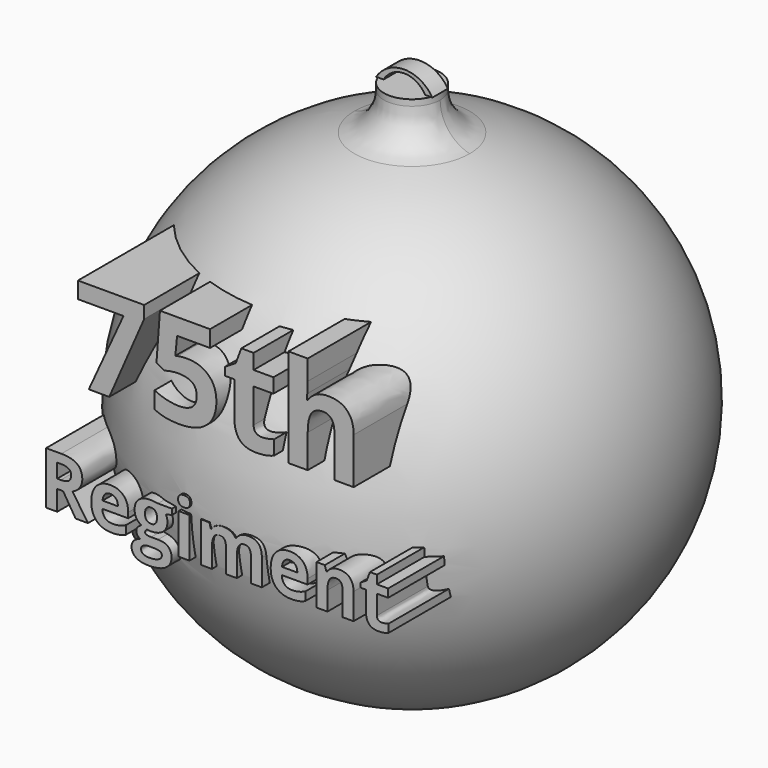
from build123d import *

# Parameters (mm, degrees)
F2_R          = 3.6879360159
F3_DEPTH      = 36.576
F4_R          = 5.08
F6_DEPTH      = 1.27
F8_DEPTH      = 12.7
F9_TEXT_SIZE  = 16.9737471475
F10_DEPTH     = 31.242
F11_TEXT_SIZE = 9.6334003123
F12_DEPTH     = 31.75


# Not quite as in the source:
# - Text() gives the source's letters only with a copy of the font that has no kerning and outlines rounded to 1/6400 em; it was checked with that copy


with BuildPart() as f1:
    # F0 (on Front) → F1 (revolve)
    with BuildSketch(Plane.XZ):
        with BuildLine():
            Line((0, -31.75), (0, 31.75))
            ThreePointArc((0, 31.75), (-31.75, 0), (0, -31.75))
        make_face()
    revolve(axis=Axis((0, 0, -12.3165734112), (0, 0, -1)))

    # F2 (on Top) → F3 (join)
    with BuildSketch(Plane.XY):
        Circle(F2_R)
    extrude(amount=F3_DEPTH)

    # F4
    f4_edges = [f1.edges().sort_by_distance(p)[0] for p in [
        (0, -3.687936, 31.535086),
        (0, 3.687936, 31.535086),
    ]]
    fillet(f4_edges, radius=F4_R)

    # F5 (on Front) → F6 (join, symmetric)
    with BuildSketch(Plane.XZ):
        with BuildLine():
            ThreePointArc((3.6879360159, 36.576), (0, 38.623130259), (-3.6879360159, 36.576))
            Line((-3.6879360159, 36.576), (3.6879360159, 36.576))
        make_face()
    extrude(amount=F6_DEPTH, both=True)

    # F7 (on Front) → F8 (cut, symmetric)
    with BuildSketch(Plane.XZ):
        with BuildLine():
            ThreePointArc((2.7261478826, 36.576), (0.0050439266, 38.170317006), (-2.7160600293, 36.576))
            Line((-2.7160600293, 36.576), (2.7261478826, 36.576))
        make_face()
    extrude(amount=F8_DEPTH, both=True, mode=Mode.SUBTRACT)

    # F9 (on Front) → F10 (join)
    with BuildSketch(Plane.XZ):
        with Locations((-19.286419265, 8.2110501826)):
            Text('75th', F9_TEXT_SIZE, font='Open Sans', font_style=FontStyle.BOLD, text_align=(TextAlign.LEFT, TextAlign.BOTTOM))
    extrude(amount=F10_DEPTH)

    # F11 (on Front) → F12 (join)
    with BuildSketch(Plane.XZ):
        with Locations((-23.4648060607, -6.9360482249)):
            Text('Regiment', F11_TEXT_SIZE, font='Open Sans', font_style=FontStyle.BOLD, text_align=(TextAlign.LEFT, TextAlign.BOTTOM))
    extrude(amount=F12_DEPTH)


solid = f1.part
